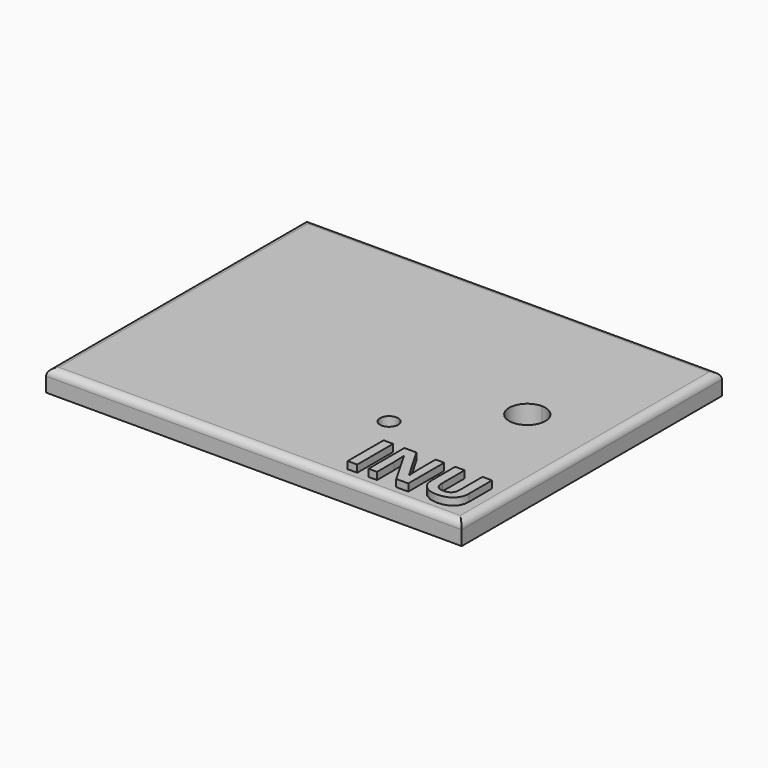
from build123d import *

# Parameters (mm, degrees)
F1_DEPTH     = 6
F2_TEXT_SIZE = 17.3875441154
F3_DEPTH     = 8
F4_R         = 2
F5_R         = 2.5
F6_DEPTH     = 10
F7_W         = 2.1
F7_H         = 2.5
F8_DEPTH     = 55


# Not quite as in the source:
# - Text() gives the source's letters only with a copy of the font that has no kerning and outlines rounded to 1/6400 em; it was checked with that copy


with BuildPart() as f1:
    # F0 (on Top) → F1 (new body)
    with BuildSketch(Plane.XY):
        Polygon((57.5, 38.1674032978), (-57.5, 38.1674032978), (-57.5, -51.8325967022), (57.5, -51.8325967022), (57.5, -33.4088504314), align=None)
    extrude(amount=F1_DEPTH)

    # F4
    f4_edges = [f1.edges().sort_by_distance(p)[0] for p in [
        (0, 38.167403, 6),
        (-57.5, -6.832597, 6),
        (0, -51.832597, 6),
        (57.5, -6.832597, 6),
    ]]
    fillet(f4_edges, radius=F4_R)

    # F5 (on face) → F6 (cut)
    with BuildSketch(Plane.XY.offset(6)):
        with BuildLine():
            Line((37.2504517436, -3.8325967022), (42.2504517436, -3.8325967022))
            ThreePointArc((42.2504517436, -3.8325967022), (40.7859856495, -0.2970627963), (37.2504517436, 1.1674032978))
            Line((37.2504517436, 1.1674032978), (37.2504517436, -3.8325967022))
        make_face()
        with BuildLine():
            ThreePointArc((37.2504517436, 1.1674032978), (33.7149178377, -7.3681306082), (42.2504517436, -3.8325967022))
            Line((42.2504517436, -3.8325967022), (37.2504517436, -3.8325967022))
            Line((37.2504517436, -3.8325967022), (37.2504517436, 1.1674032978))
        make_face()
        with Locations((16.0049460828, -25.0696968287)):
            Circle(F5_R)
    extrude(amount=-F6_DEPTH, mode=Mode.SUBTRACT)

    # F7 (on Right) → F8 (cut, symmetric)
    with BuildSketch(Plane.YZ):
        with Locations((36.8532956719, 1.25)):
            Rectangle(F7_W, F7_H)
    extrude(amount=F8_DEPTH, both=True, mode=Mode.SUBTRACT)


with BuildPart() as f3:
    # F2 (on face) → F3 (new body)
    with BuildSketch(Plane.XY):
        with Locations((21.4203363284, -48.115812242)):
            Text('INU', F2_TEXT_SIZE, font='Open Sans', font_style=FontStyle.BOLD, text_align=(TextAlign.LEFT, TextAlign.BOTTOM))
    extrude(amount=F3_DEPTH)


solid = Compound([f1.part, f3.part])
